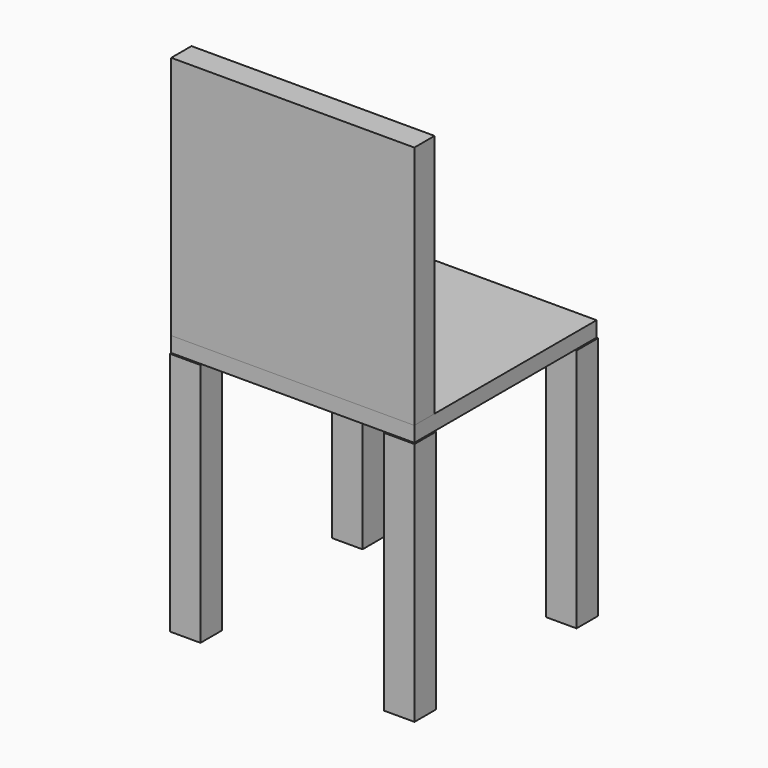
from build123d import *

# Parameters (mm, degrees)
F1_DEPTH = 406.4
F0_W     = 50.8
F0_H     = 44.8537981102
F2_W     = 50.8
F2_H     = 44.8537981102
F3_DEPTH = 25.4
F4_W     = 403.8771986961
F4_H     = 42.064961046
F5_DEPTH = 406.4


# Not quite as in the source:
# - a feature names something its author has since deleted; it is built from what else it names


with BuildPart() as f1:
    # F0 (on Top) → F1 (new body)
    with BuildSketch(Plane.XY):
        Polygon((50.8, 0), (0, 0), (0, -44.8537981102), (50.8, -44.8537981102), (50.8, -22.4268990551), align=None)
    extrude(amount=F1_DEPTH)


with BuildPart() as f1b:
    # F0 (on Top) → F1, piece 2 (new body)
    with BuildSketch(Plane.XY):
        with Locations((381, 314.1055959259)):
            Rectangle(F0_W, F0_H)
    extrude(amount=F1_DEPTH)


with BuildPart() as f1c:
    # F0 (on Top) → F1, piece 3 (new body)
    with BuildSketch(Plane.XY):
        Polygon((355.6, 0), (355.6, -22.4268990551), (355.6, -44.8537981102), (406.4, -44.8537981102), (406.4, 0), align=None)
    extrude(amount=F1_DEPTH)


with BuildPart() as f1d:
    # F0 (on Top) → F1, piece 4 (new body)
    with BuildSketch(Plane.XY):
        with Locations((25.4, 314.1055959259)):
            Rectangle(F0_W, F0_H)
    extrude(amount=F1_DEPTH)


with BuildPart() as f3:
    # F2 (on face) → F3 (new body)
    with BuildSketch(Plane.XY.offset(406.4)):
        Polygon((50.8, 291.6786968708), (0, 291.6786968708), (0, -42.064961046), (403.8771986961, -42.064961046), (403.8771986961, 336.532494981), (50.8, 336.532494981), align=None)
        with Locations((25.4, 314.1055959259)):
            Rectangle(F2_W, F2_H)
    extrude(amount=F3_DEPTH)


with BuildPart() as f5:
    # F4 (on face) → F5 (new body)
    with BuildSketch(Plane.XY.offset(431.8)):
        with Locations((201.9385993481, -21.032480523)):
            Rectangle(F4_W, F4_H)
    extrude(amount=F5_DEPTH)


solid = Compound([f1.part, f1b.part, f1c.part, f1d.part, f3.part, f5.part])
